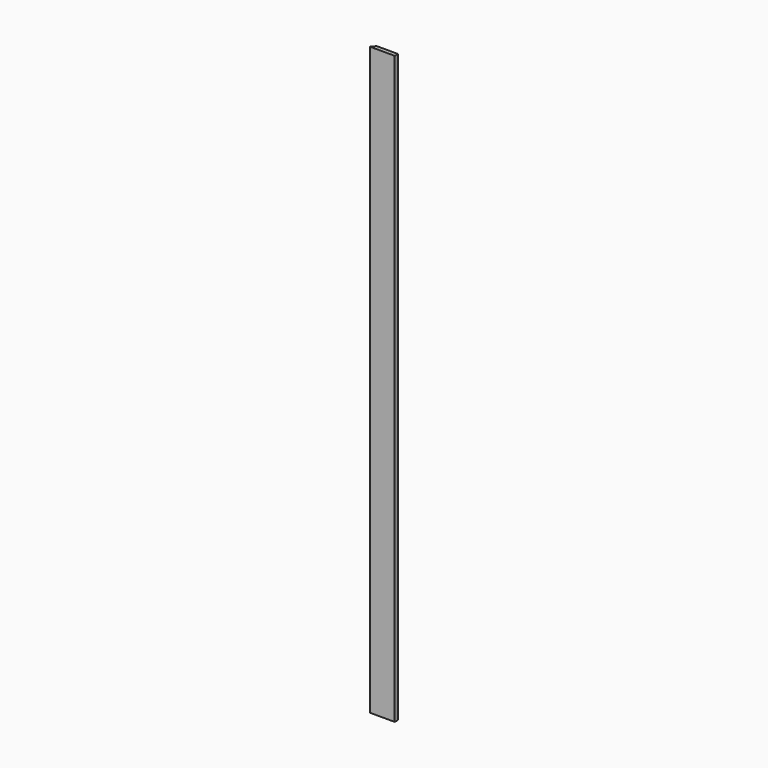
from build123d import *

# Parameters (mm, degrees)
F1_DEPTH = 457.2


with BuildPart() as f1:
    # F0 (on Top) → F1 (new body)
    with BuildSketch(Plane.XY):
        Polygon((-2.664141329, 0), (0, 0), (1.6153912187, 0), (16.6282931011, 0), (16.6282931011, 3.175), (0, 3.175), align=None)
    extrude(amount=F1_DEPTH)


solid = f1.part
